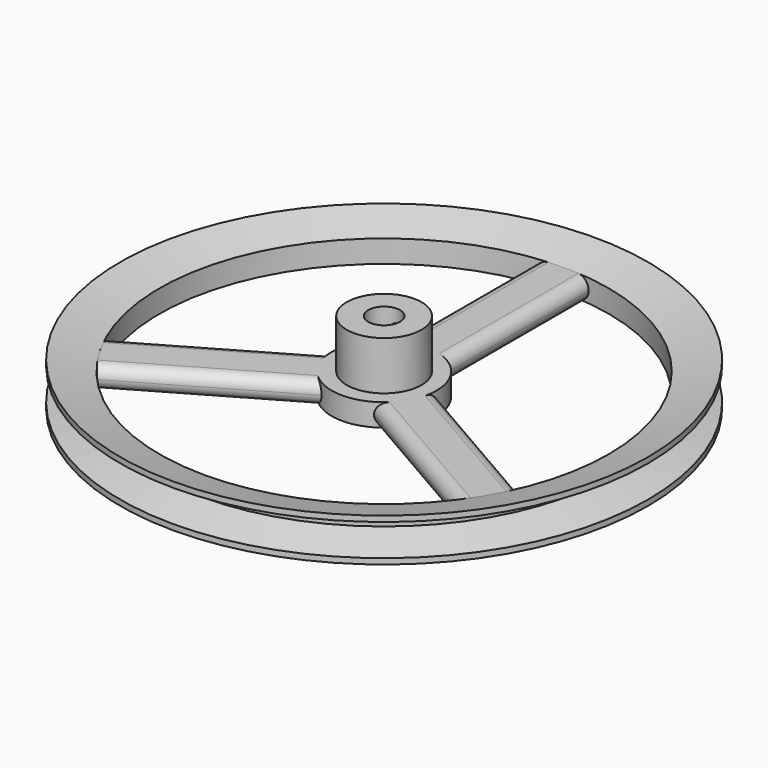
from build123d import *

# Parameters (mm, degrees)
F0_R          = 141
F0_R_2        = 120
F1_DEPTH      = 11.5
F7_DEPTH      = 6
F8_R          = 20
F9_DEPTH      = 26
F9_DEPTH_BACK = 14
F10_R         = 8.5
F11_DEPTH     = 43.501
F12_R         = 5.99999
F13_R         = 3
F14_DEPTH     = 141.001


# Not quite as in the source:
# - a fillet or chamfer is up to 0.001 mm smaller than in the source, because OpenCascade refuses the exact size


with BuildPart() as f1:
    # F0 (on Top) → F1 (new body, symmetric)
    with BuildSketch(Plane.XY):
        Circle(F0_R)
        Circle(F0_R_2, mode=Mode.SUBTRACT)
    extrude(amount=F1_DEPTH, both=True)

    # F2 (on Right) → F3 (revolve, cut)
    with BuildSketch(Plane.YZ):
        Polygon((-122, 3.5), (-141, 8.5), (-141, -8.5), (-122, -3.5), align=None)
    revolve(axis=Axis((0, 0, 28.2399164939), (0, 0, 1)), mode=Mode.SUBTRACT)

    # F4 (on Right) → F5 (revolve, cut)
    with BuildSketch(Plane.YZ):
        Polygon((-141, 11.5), (-120, 6), (-120, 11.5), align=None)
        Polygon((-120, -6), (-141, -11.5), (-120, -11.5), align=None)
    revolve(axis=Axis((0, 0, 29.001140967), (0, 0, 1)), mode=Mode.SUBTRACT)


with BuildPart() as f7:
    # F6 (on Top) → F7 (new body, symmetric)
    with BuildSketch(Plane.XY):
        with BuildLine():
            Line((-14, 119.1805353235), (-14, 24.248711306))
            ThreePointArc((-14, 24.248711306), (-24.248711306, 14), (-28, 0))
            Line((-28, 0), (-110.2133712268, -47.4659120088))
            ThreePointArc((-110.2133712268, -47.4659120088), (-103.9230484541, -60), (-96.2133712268, -71.7146233147))
            Line((-96.2133712268, -71.7146233147), (-14, -24.248711306))
            ThreePointArc((-14, -24.248711306), (0, -28), (14, -24.248711306))
            Line((14, -24.248711306), (96.2133712268, -71.7146233147))
            ThreePointArc((96.2133712268, -71.7146233147), (103.9230484541, -60), (110.2133712268, -47.4659120088))
            Line((110.2133712268, -47.4659120088), (28, 0))
            ThreePointArc((28, 0), (24.248711306, 14), (14, 24.248711306))
            Line((14, 24.248711306), (14, 119.1805353235))
            ThreePointArc((14, 119.1805353235), (0, 120), (-14, 119.1805353235))
        make_face()
    extrude(amount=F7_DEPTH, both=True)

    # F8 (on face) → F9 (join, two sides)
    with BuildSketch(Plane.XY.offset(6)) as f9_sk:
        Circle(F8_R)
    extrude(amount=F9_DEPTH)
    extrude(f9_sk.sketch, amount=-F9_DEPTH_BACK)

    # F10 (on face) → F11 (cut, through all)
    with BuildSketch(Plane.XY.offset(32)):
        Circle(F10_R)
    extrude(amount=-F11_DEPTH, mode=Mode.SUBTRACT)

    # F12 (radius 6 in the source; OpenCascade refuses exactly that, so slightly less here)
    f12_edges = [f7.edges().sort_by_distance(p)[0] for p in [
        (-14, 71.714623, 6),
        (-14, 71.714623, -6),
        (14, 71.714623, 6),
        (14, 71.714623, -6),
        (69.106686, -23.732956, -6),
        (69.106686, -23.732956, 6),
        (55.106686, -47.981667, 6),
        (55.106686, -47.981667, -6),
        (-55.106686, -47.981667, 6),
        (-55.106686, -47.981667, -6),
        (-69.106686, -23.732956, 6),
        (-69.106686, -23.732956, -6),
    ]]
    fillet(f12_edges, radius=F12_R)

    # F13 (on Front) → F14 (cut, through all)
    with BuildSketch(Plane.XZ):
        with Locations((0, 22)):
            Circle(F13_R)
    extrude(amount=-F14_DEPTH, mode=Mode.SUBTRACT)


solid = Compound([f1.part, f7.part])
